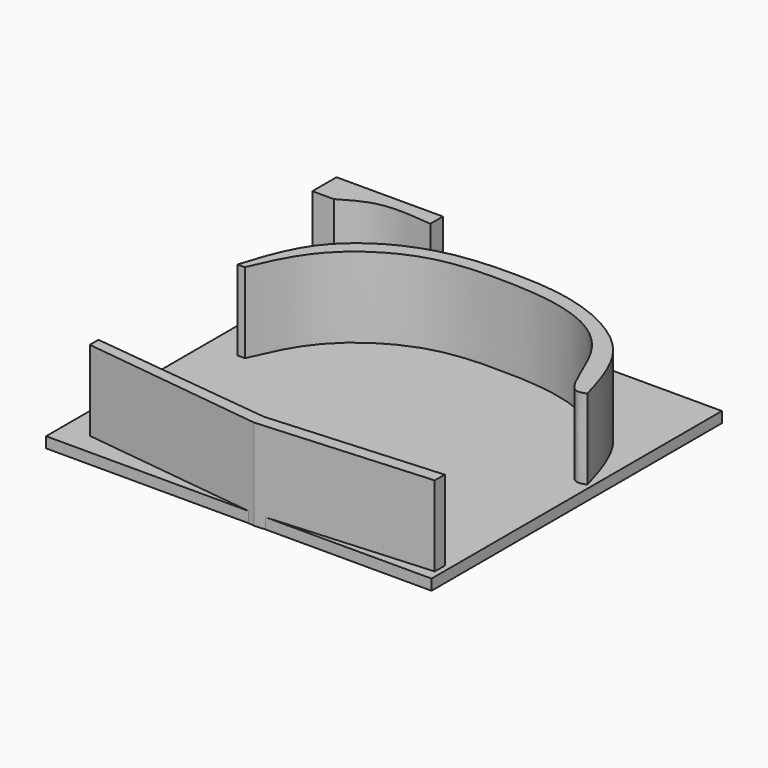
from build123d import *

# Parameters (mm, degrees)
F2_DEPTH = 25.4
F4_DEPTH = 25.4
F7_W     = 107.728920877
F7_H     = 101.4381758869
F8_DEPTH = 3


# Not quite as in the source:
# - a feature of the source that left no trace in its solid (it failed there, or was rolled back) is left out


with BuildPart() as f2:
    # F1 (on Top) → F2 (new body)
    with BuildSketch(Plane.XY):
        Polygon((0, -52.5968633592), (-50.9308427572, -46.761199832), (-50.9308427572, -49.7846864164), (0, -56.0923367739), (47.871535476, -52.812457282), (47.9106865823, -49.314301461), align=None)
    extrude(amount=F2_DEPTH)


with BuildPart() as f2b:
    # F1 (on Top) → F2, piece 2 (new body)
    with BuildSketch(Plane.XY):
        with BuildLine():
            add(Edge.make_bspline(
                [(-49.4719222188, 0), (-47.4205755879, 6.544775019), (-43.1942210623, 20.0288635212), (-22.5111385572, 33.2669128259), (0.0334513522, 34.6754363871), (20.6787838864, 33.2616809804), (42.0254177462, 21.7261812452), (46.1992146547, 7.2172589855), (48.275411129, 0)],
                knots=[0, 0, 0, 0, 0.1613126113, 0.3323496255, 0.5013055914, 0.6641099851, 0.8329162439, 1, 1, 1, 1], degree=3))
            add(Edge.make_bspline(
                [(-49.4719222188, 0), (-48.7881400085, 0), (-48.1043577982, 0), (-47.4205755879, 0)],
                knots=[0, 0, 0, 0, 2.0513466309, 2.0513466309, 2.0513466309, 2.0513466309], degree=3))
            add(Edge.make_bspline(
                [(-47.4205755879, 0), (-45.023795475, 5.5050731836), (-40.013610592, 17.0127764963), (-20.8333104147, 29.7676194141), (-0.1210192078, 30.7096554729), (21.0037992002, 29.3354980818), (37.8639372795, 19.2664559838), (43.1661496501, -1.7953891308), (47.0887209969, -0.4170016691), (48.275411129, 0)],
                knots=[0, 0, 0, 0, 0.1491588243, 0.3117988516, 0.4707933547, 0.6300285532, 0.78410953, 0.9346869521, 1, 1, 1, 1], degree=3))
        make_face()
    extrude(amount=F2_DEPTH)


with BuildPart() as f4:
    # F0 (on Top) → F4 (new body)
    with BuildSketch(Plane.XY):
        with BuildLine():
            Line((-58.3559162915, 37.2523628175), (-52.3617714643, 37.2523628175))
            add(Edge.make_bspline(
                [(-52.3617714643, 37.2523628175), (-49.4308542357, 38.9942348261), (-43.0485284896, 42.7873117707), (-33.688896908, 41.8152382446), (-28.6274328828, 41.2895642221)],
                knots=[0, 0, 0, 0, 0.459224011, 1, 1, 1, 1], degree=3))
            Line((-28.6274328828, 41.2895642221), (-28.6274328828, 45.6937812269))
            Line((-28.6274328828, 45.6937812269), (-58.3559162915, 45.6937812269))
            Line((-58.3559162915, 45.6937812269), (-58.3559162915, 37.2523628175))
        make_face()
    extrude(amount=F4_DEPTH)


with BuildPart() as f8:
    # F7 (on Top) → F8 (new body)
    with BuildSketch(Plane.XY):
        with Locations((-4.40428406, -5.1615331322)):
            Rectangle(F7_W, F7_H)
    extrude(amount=F8_DEPTH)


solid = Compound([f2.part, f2b.part, f4.part, f8.part])
